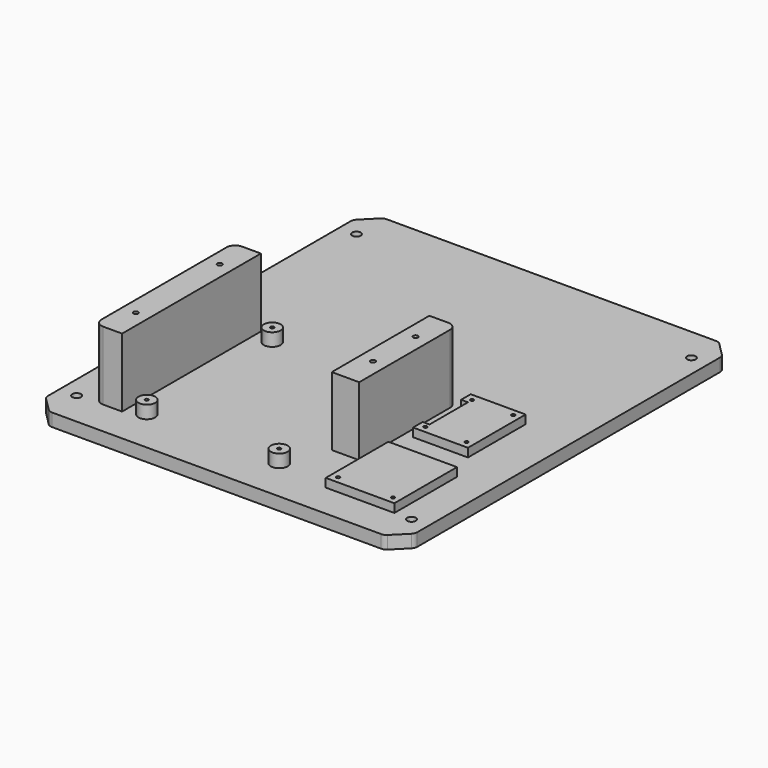
from build123d import *

# Parameters (mm, degrees)
F4_W      = 136.645
F4_H      = 154.85
F5_DEPTH  = 4.7625
F0_R      = 3.1
F0_R_2    = 1.375
F6_DEPTH  = 4.7625
F7_DEPTH  = 25.4
F3_R      = 1.143
F8_DEPTH  = 3.175
F2_W      = 25.4
F2_H      = 28.956
F2_R      = 1.143
F9_DEPTH  = 3.175
F10_R     = 0.635
F11_DEPTH = 7.62
F12_R     = 0.635
F14_DEPTH = 7.62
F15_R     = 0.889
F16_DEPTH = 25.4
F17_SIZE  = 6.35
F18_R     = 2.54
F19_R     = 1.5875
F20_DEPTH = 4.7635


# Not quite as in the source:
# - a feature names something its author has since deleted; it is built from what else it names


with BuildPart() as f5:
    # F4 (on Top) → F5 (new body)
    with BuildSketch(Plane.XY):
        with Locations((14.2875, 26.225)):
            Rectangle(F4_W, F4_H)
    extrude(amount=-F5_DEPTH)

    # F0 (on Top) → F6 (join)
    with BuildSketch(Plane.XY):
        with Locations((-24.5, 23)):
            Circle(F0_R)
        with Locations((-24.5, 23)):
            Circle(F0_R_2, mode=Mode.SUBTRACT)
        with Locations((24.5, 23)):
            Circle(F0_R)
        with Locations((24.5, 23)):
            Circle(F0_R_2, mode=Mode.SUBTRACT)
        with Locations((-24.5, -35)):
            Circle(F0_R)
        with Locations((-24.5, -35)):
            Circle(F0_R_2, mode=Mode.SUBTRACT)
        with Locations((24.5, -35)):
            Circle(F0_R)
        with Locations((24.5, -35)):
            Circle(F0_R_2, mode=Mode.SUBTRACT)
        with Locations((-24.5, 23)):
            Circle(F0_R_2)
        with Locations((24.5, 23)):
            Circle(F0_R_2)
        with Locations((-24.5, -35)):
            Circle(F0_R_2)
        with Locations((24.5, -35)):
            Circle(F0_R_2)
    extrude(amount=F6_DEPTH)

    # F1 (on Top) → F7 (join)
    with BuildSketch(Plane.XY):
        with BuildLine():
            ThreePointArc((-41.335, -34.925), (-40.4050640303, -37.1700640303), (-38.16, -38.1))
            Line((-38.16, -38.1), (-34.35, -38.1))
            Line((-34.35, -38.1), (-31.175, -38.1))
            Line((-31.175, -38.1), (-31.175, -34.925))
            Line((-31.175, -34.925), (-31.175, 22.925))
            Line((-31.175, 22.925), (-31.175, 26.1))
            Line((-31.175, 26.1), (-38.16, 26.1))
            ThreePointArc((-38.16, 26.1), (-40.4050640303, 25.1700640303), (-41.335, 22.925))
            Line((-41.335, 22.925), (-41.335, -34.925))
        make_face()
        with BuildLine():
            Line((31.175, 26.1), (31.175, 22.925))
            Line((31.175, 22.925), (31.175, -19.05))
            Line((31.175, -19.05), (41.335, -19.05))
            Line((41.335, -19.05), (41.335, 22.925))
            ThreePointArc((41.335, 22.925), (40.4050640303, 25.1700640303), (38.16, 26.1))
            Line((38.16, 26.1), (31.175, 26.1))
        make_face()
    extrude(amount=F7_DEPTH)

    # F3 (on Top) → F8 (join)
    with BuildSketch(Plane.XY):
        Polygon((64.83, 28.556), (44.51, 28.556), (44.51, 24.111), (47.05, 24.111), (47.05, 6.331), (44.51, 6.331), (44.51, 1.886), (64.83, 1.886), align=None)
        with Locations((47.05, 4.426)):
            Circle(F3_R, mode=Mode.SUBTRACT)
        with Locations((62.29, 4.426)):
            Circle(F3_R, mode=Mode.SUBTRACT)
        with Locations((47.05, 26.016)):
            Circle(F3_R, mode=Mode.SUBTRACT)
        with Locations((62.29, 26.016)):
            Circle(F3_R, mode=Mode.SUBTRACT)
        with Locations((62.29, 4.426)):
            Circle(F3_R)
        with Locations((62.29, 26.016)):
            Circle(F3_R)
        with Locations((47.05, 26.016)):
            Circle(F3_R)
        with Locations((47.05, 4.426)):
            Circle(F3_R)
    extrude(amount=F8_DEPTH)

    # F2 (on Top) → F9 (join)
    with BuildSketch(Plane.XY):
        with Locations((57.21, -24.022)):
            Rectangle(F2_W, F2_H)
        with Locations((47.05, -35.96)):
            Circle(F2_R, mode=Mode.SUBTRACT)
        with Locations((67.37, -35.96)):
            Circle(F2_R, mode=Mode.SUBTRACT)
        with Locations((47.05, -35.96)):
            Circle(F2_R)
        with Locations((67.37, -35.96)):
            Circle(F2_R)
    extrude(amount=F9_DEPTH)

    # F10 (on face) → F11 (cut)
    with BuildSketch(Plane.XY.offset(3.175)):
        with Locations((47.05, 26.016)):
            Circle(F10_R)
        with Locations((62.29, 26.016)):
            Circle(F10_R)
        with Locations((62.29, 4.426)):
            Circle(F10_R)
        with Locations((47.05, 4.426)):
            Circle(F10_R)
        with Locations((47.05, -35.96)):
            Circle(F10_R)
        with Locations((67.37, -35.96)):
            Circle(F10_R)
    extrude(amount=-F11_DEPTH, mode=Mode.SUBTRACT)

    # F12 (on face) → F14 (cut)
    with BuildSketch(Plane.XY.offset(4.7625)):
        with Locations((-24.5, 23)):
            Circle(F12_R)
        with Locations((24.5, 23)):
            Circle(F12_R)
        with Locations((24.5, -35)):
            Circle(F12_R)
        with Locations((-24.5, -35)):
            Circle(F12_R)
    extrude(amount=-F14_DEPTH, mode=Mode.SUBTRACT)

    # F15 (on face) → F16 (cut)
    with BuildSketch(Plane.XY.offset(25.4)):
        with Locations((-36.255, 13.4)):
            Circle(F15_R)
        with Locations((36.255, -6.35)):
            Circle(F15_R)
        with Locations((36.255, 13.4)):
            Circle(F15_R)
        with Locations((-36.255, -25.4)):
            Circle(F15_R)
    extrude(amount=-F16_DEPTH, mode=Mode.SUBTRACT)

    # F17
    f17_edges = [f5.edges().sort_by_distance(p)[0] for p in [
        (-54.035, 103.65, -2.38125),
        (82.61, 103.65, -2.38125),
        (82.61, -51.2, -2.38125),
        (-54.035, -51.2, -2.38125),
    ]]
    chamfer(f17_edges, length=F17_SIZE)

    # F18
    f18_edges = [f5.edges().sort_by_distance(p)[0] for p in [
        (82.61, 97.3, -2.38125),
        (76.26, 103.65, -2.38125),
        (-47.685, 103.65, -2.38125),
        (-54.035, 97.3, -2.38125),
        (-54.035, -44.85, -2.38125),
        (-47.685, -51.2, -2.38125),
        (76.26, -51.2, -2.38125),
        (82.61, -44.85, -2.38125),
    ]]
    fillet(f18_edges, radius=F18_R)

    # F19 (on face) → F20 (cut, through all)
    with BuildSketch(Plane.XY):
        with Locations((-47.685, 90.95)):
            Circle(F19_R)
        with Locations((76.26, 90.95)):
            Circle(F19_R)
        with Locations((76.26, -38.5)):
            Circle(F19_R)
        with Locations((-47.685, -38.5)):
            Circle(F19_R)
    extrude(amount=-F20_DEPTH, mode=Mode.SUBTRACT)


solid = f5.part
